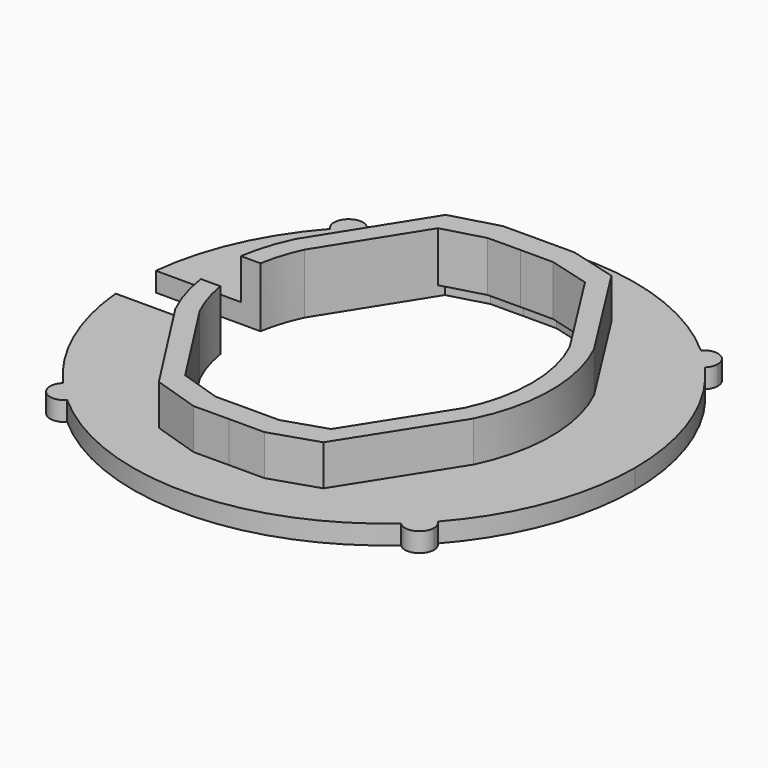
from build123d import *

# Parameters (mm, degrees)
F1_DEPTH = 3.1
F3_DEPTH = 1
F5_DEPTH = 3.1
F7_DEPTH = 2.6


# Not quite as in the source:
# - ends of sketch curves that miss each other by under 0.0002 mm in the source are joined


with BuildPart() as f1:
    # F0 (on Top) → F1 (new body)
    with BuildSketch(Plane.XY):
        with BuildLine():
            Line((-45.1821846682, -49.2377741688), (-48.6372292437, -43.7981166044))
            Line((-48.6372292437, -43.7981166044), (-51.0690886894, -43.1337059986))
            Line((-51.0690886894, -43.1337059986), (-52.9226313652, -43.1337059986))
            Line((-52.9226313652, -43.1337059986), (-54.7761512226, -43.1429032238))
            Line((-54.7761512226, -43.1429032238), (-57.2046839443, -43.8193724666))
            Line((-57.2046839443, -43.8193724666), (-60.6326945623, -49.2761068966))
            ThreePointArc((-60.6326945623, -49.2761068966), (-61.5175196788, -53.1892877339), (-60.5939044307, -57.0934950318))
            Line((-60.5939044307, -57.0934950318), (-57.1270457212, -62.4923727119))
            Line((-57.1270457212, -62.4923727119), (-54.7013924586, -63.2718429691))
            Line((-54.7013924586, -63.2718429691), (-52.8726911435, -63.2627688943))
            Line((-52.8726911435, -63.2627688943), (-51.0439673156, -63.2627688943))
            Line((-51.0439673156, -63.2627688943), (-48.6222116233, -62.4712722115))
            Line((-48.6222116233, -62.4712722115), (-45.1821846682, -57.0552585424))
            ThreePointArc((-45.1821846682, -57.0552585424), (-44.2779533541, -53.1465163556), (-45.1821846682, -49.2377741688))
        make_face()
        with BuildLine():
            Line((-51.2032357795, -44.1337052485), (-49.2739452053, -44.6608085404))
            Line((-49.2739452053, -44.6608085404), (-46.0570379398, -49.725540285))
            ThreePointArc((-46.0570379398, -49.725540285), (-45.277952604, -53.1465163556), (-46.0570379398, -56.5674924262))
            Line((-46.0570379398, -56.5674924262), (-49.2739452053, -61.6322241709))
            Line((-49.2739452053, -61.6322241709), (-51.2032357795, -62.2627696444))
            Line((-51.2032357795, -62.2627696444), (-52.8751721425, -62.2627696444))
            Line((-52.8751721425, -62.2627696444), (-54.5470879228, -62.2710657443))
            Line((-54.5470879228, -62.2710657443), (-56.4794834946, -61.6501011173))
            Line((-56.4794834946, -61.6501011173), (-59.7214822105, -56.6013939237))
            ThreePointArc((-59.7214822105, -56.6013939237), (-60.5175327396, -53.1843257665), (-59.7554317793, -49.7595260114))
            Line((-59.7554317793, -49.7595260114), (-56.5636951686, -44.678894416))
            Line((-56.5636951686, -44.678894416), (-54.6370438166, -44.1422245291))
            Line((-54.6370438166, -44.1422245291), (-52.9201503662, -44.1337052485))
            Line((-52.9201503662, -44.1337052485), (-51.2032357795, -44.1337052485))
        make_face(mode=Mode.SUBTRACT)
    extrude(amount=F1_DEPTH)

    # F2 (on face) → F3 (join)
    with BuildSketch(Plane(origin=(0, 0, 0), x_dir=(1, 0, 0), z_dir=(0, 0, -1))):
        with BuildLine():
            ThreePointArc((-43.358584194, 62.0303384897), (-43.2740778057, 61.9381826183), (-43.1904616862, 61.8452182226))
            ThreePointArc((-43.1904616862, 61.8452182226), (-43.0165755747, 62.0936479592), (-42.9552730989, 62.3906256019))
            ThreePointArc((-42.9552730989, 62.3906256019), (-43.4282853143, 63.0876031964), (-44.2506804781, 62.9054370146))
            ThreePointArc((-44.2506804781, 62.9054370146), (-44.1577160825, 62.8218208951), (-44.0655602111, 62.7373145068))
            ThreePointArc((-44.0655602111, 62.7373145068), (-43.5183821629, 62.8543839205), (-43.2052730989, 62.3906256019))
            ThreePointArc((-43.2052730989, 62.3906256019), (-43.2451945988, 62.1948507981), (-43.358584194, 62.0303384897))
        make_face()
        with BuildLine():
            ThreePointArc((-44.0655602111, 62.7373145068), (-43.7052730989, 62.3906256019), (-43.358584194, 62.0303384897))
            ThreePointArc((-43.358584194, 62.0303384897), (-43.2451945988, 62.1948507981), (-43.2052730989, 62.3906256019))
            ThreePointArc((-43.2052730989, 62.3906256019), (-43.5183821629, 62.8543839205), (-44.0655602111, 62.7373145068))
        make_face()
        with BuildLine():
            ThreePointArc((-44.0655602111, 62.7373145068), (-44.0588264895, 62.0370722113), (-43.358584194, 62.0303384897))
            ThreePointArc((-43.358584194, 62.0303384897), (-43.7052730989, 62.3906256019), (-44.0655602111, 62.7373145068))
        make_face()
        with BuildLine():
            ThreePointArc((-43.1904616862, 44.5512566703), (-40.748719029, 48.5718778834), (-39.8976612543, 53.1982374465))
            ThreePointArc((-39.8976612543, 53.1982374465), (-40.748719029, 57.8245970095), (-43.1904616862, 61.8452182226))
            ThreePointArc((-43.1904616862, 61.8452182226), (-44.2356031848, 61.860295516), (-44.2506804781, 62.9054370146))
            ThreePointArc((-44.2506804781, 62.9054370146), (-52.8976612543, 66.1982374465), (-61.5446420305, 62.9054370146))
            ThreePointArc((-61.5446420305, 62.9054370146), (-61.3930718153, 62.6676133864), (-61.3400494097, 62.3906256019))
            ThreePointArc((-61.3400494097, 62.3906256019), (-61.7930717671, 61.7019280777), (-62.6048608225, 61.8452182226))
            ThreePointArc((-62.6048608225, 61.8452182226), (-65.8976612543, 53.1982374465), (-62.6048608225, 44.5512566703))
            ThreePointArc((-62.6048608225, 44.5512566703), (-61.7930717671, 44.6945468152), (-61.3400494097, 44.005849291))
            ThreePointArc((-61.3400494097, 44.005849291), (-61.3930718153, 43.7288615065), (-61.5446420305, 43.4910378783))
            ThreePointArc((-61.5446420305, 43.4910378783), (-52.8976612543, 40.1982374465), (-44.2506804781, 43.4910378783))
            ThreePointArc((-44.2506804781, 43.4910378783), (-44.2356031848, 44.5361793769), (-43.1904616862, 44.5512566703))
        make_face()
        with BuildLine():
            Line((-45.1821846682, 49.2377741688), (-48.6372292437, 43.7981166044))
            Line((-48.6372292437, 43.7981166044), (-51.0690886894, 43.1337059986))
            Line((-51.0690886894, 43.1337059986), (-52.9226313652, 43.1337059986))
            Line((-52.9226313652, 43.1337059986), (-54.7761512226, 43.1429032238))
            Line((-54.7761512226, 43.1429032238), (-57.2046839443, 43.8193724666))
            Line((-57.2046839443, 43.8193724666), (-60.6326945623, 49.2761068966))
            ThreePointArc((-60.6326945623, 49.2761068966), (-61.5175196788, 53.1892877339), (-60.5939044307, 57.0934950318))
            Line((-60.5939044307, 57.0934950318), (-57.1270457212, 62.4923727119))
            Line((-57.1270457212, 62.4923727119), (-54.7013924586, 63.2718429691))
            Line((-54.7013924586, 63.2718429691), (-52.8726911435, 63.2627688943))
            Line((-52.8726911435, 63.2627688943), (-51.0439673156, 63.2627688943))
            Line((-51.0439673156, 63.2627688943), (-48.6222116233, 62.4712722115))
            Line((-48.6222116233, 62.4712722115), (-45.1821846682, 57.0552585424))
            ThreePointArc((-45.1821846682, 57.0552585424), (-44.2779533541, 53.1465163556), (-45.1821846682, 49.2377741688))
        make_face(mode=Mode.SUBTRACT)
        with BuildLine():
            ThreePointArc((-44.2506804781, 62.9054370146), (-44.2356031848, 61.860295516), (-43.1904616862, 61.8452182226))
            ThreePointArc((-43.1904616862, 61.8452182226), (-43.2740778057, 61.9381826183), (-43.358584194, 62.0303384897))
            ThreePointArc((-43.358584194, 62.0303384897), (-44.0588264895, 62.0370722113), (-44.0655602111, 62.7373145068))
            ThreePointArc((-44.0655602111, 62.7373145068), (-44.1577160825, 62.8218208951), (-44.2506804781, 62.9054370146))
        make_face()
        with BuildLine():
            ThreePointArc((-61.7297622975, 62.7373145068), (-61.6376064262, 62.8218208951), (-61.5446420305, 62.9054370146))
            ThreePointArc((-61.5446420305, 62.9054370146), (-62.6203794956, 62.9209556878), (-62.6048608225, 61.8452182226))
            ThreePointArc((-62.6048608225, 61.8452182226), (-62.521244703, 61.9381826183), (-62.4367383146, 62.0303384897))
            ThreePointArc((-62.4367383146, 62.0303384897), (-62.4436028003, 62.7441789925), (-61.7297622975, 62.7373145068))
        make_face()
        with BuildLine():
            ThreePointArc((-61.3400494097, 62.3906256019), (-61.3930718153, 62.6676133864), (-61.5446420305, 62.9054370146))
            ThreePointArc((-61.5446420305, 62.9054370146), (-61.6376064262, 62.8218208951), (-61.7297622975, 62.7373145068))
            ThreePointArc((-61.7297622975, 62.7373145068), (-61.6262910912, 62.5775165378), (-61.5900494097, 62.3906256019))
            ThreePointArc((-61.5900494097, 62.3906256019), (-61.894274606, 61.9305471018), (-62.4367383146, 62.0303384897))
            ThreePointArc((-62.4367383146, 62.0303384897), (-62.521244703, 61.9381826183), (-62.6048608225, 61.8452182226))
            ThreePointArc((-62.6048608225, 61.8452182226), (-61.7930717671, 61.7019280777), (-61.3400494097, 62.3906256019))
        make_face()
        with BuildLine():
            ThreePointArc((-62.4367383146, 62.0303384897), (-62.0900494097, 62.3906256019), (-61.7297622975, 62.7373145068))
            ThreePointArc((-61.7297622975, 62.7373145068), (-62.4436028003, 62.7441789925), (-62.4367383146, 62.0303384897))
        make_face()
        with BuildLine():
            ThreePointArc((-61.5900494097, 62.3906256019), (-61.6262910912, 62.5775165378), (-61.7297622975, 62.7373145068))
            ThreePointArc((-61.7297622975, 62.7373145068), (-62.0900494097, 62.3906256019), (-62.4367383146, 62.0303384897))
            ThreePointArc((-62.4367383146, 62.0303384897), (-61.894274606, 61.9305471018), (-61.5900494097, 62.3906256019))
        make_face()
        with BuildLine():
            ThreePointArc((-42.9552730989, 44.005849291), (-43.0165755747, 44.3028269337), (-43.1904616862, 44.5512566703))
            ThreePointArc((-43.1904616862, 44.5512566703), (-43.2740778057, 44.4582922746), (-43.358584194, 44.3661364032))
            ThreePointArc((-43.358584194, 44.3661364032), (-43.2451945988, 44.2016240948), (-43.2052730989, 44.005849291))
            ThreePointArc((-43.2052730989, 44.005849291), (-43.5183821629, 43.5420909724), (-44.0655602111, 43.6591603861))
            ThreePointArc((-44.0655602111, 43.6591603861), (-44.1577160825, 43.5746539978), (-44.2506804781, 43.4910378783))
            ThreePointArc((-44.2506804781, 43.4910378783), (-43.4282853143, 43.3088716965), (-42.9552730989, 44.005849291))
        make_face()
        with BuildLine():
            ThreePointArc((-43.2052730989, 44.005849291), (-43.2451945988, 44.2016240948), (-43.358584194, 44.3661364032))
            ThreePointArc((-43.358584194, 44.3661364032), (-43.7052730989, 44.005849291), (-44.0655602111, 43.6591603861))
            ThreePointArc((-44.0655602111, 43.6591603861), (-43.5183821629, 43.5420909724), (-43.2052730989, 44.005849291))
        make_face()
        with BuildLine():
            ThreePointArc((-44.0655602111, 43.6591603861), (-43.7052730989, 44.005849291), (-43.358584194, 44.3661364032))
            ThreePointArc((-43.358584194, 44.3661364032), (-44.0588264895, 44.3594026816), (-44.0655602111, 43.6591603861))
        make_face()
        with BuildLine():
            ThreePointArc((-43.358584194, 44.3661364032), (-43.2740778057, 44.4582922746), (-43.1904616862, 44.5512566703))
            ThreePointArc((-43.1904616862, 44.5512566703), (-44.2356031848, 44.5361793769), (-44.2506804781, 43.4910378783))
            ThreePointArc((-44.2506804781, 43.4910378783), (-44.1577160825, 43.5746539978), (-44.0655602111, 43.6591603861))
            ThreePointArc((-44.0655602111, 43.6591603861), (-44.0588264895, 44.3594026816), (-43.358584194, 44.3661364032))
        make_face()
        with BuildLine():
            ThreePointArc((-62.6048608225, 44.5512566703), (-62.6203794956, 43.4755192051), (-61.5446420305, 43.4910378783))
            ThreePointArc((-61.5446420305, 43.4910378783), (-61.6376064262, 43.5746539978), (-61.7297622975, 43.6591603861))
            ThreePointArc((-61.7297622975, 43.6591603861), (-62.4436028003, 43.6522959004), (-62.4367383146, 44.3661364032))
            ThreePointArc((-62.4367383146, 44.3661364032), (-62.521244703, 44.4582922746), (-62.6048608225, 44.5512566703))
        make_face()
        with BuildLine():
            ThreePointArc((-62.4367383146, 44.3661364032), (-62.4436028003, 43.6522959004), (-61.7297622975, 43.6591603861))
            ThreePointArc((-61.7297622975, 43.6591603861), (-62.0900494097, 44.005849291), (-62.4367383146, 44.3661364032))
        make_face()
        with BuildLine():
            ThreePointArc((-62.4367383146, 44.3661364032), (-62.0900494097, 44.005849291), (-61.7297622975, 43.6591603861))
            ThreePointArc((-61.7297622975, 43.6591603861), (-61.6262910912, 43.8189583551), (-61.5900494097, 44.005849291))
            ThreePointArc((-61.5900494097, 44.005849291), (-61.894274606, 44.4659277911), (-62.4367383146, 44.3661364032))
        make_face()
        with BuildLine():
            ThreePointArc((-61.7297622975, 43.6591603861), (-61.6376064262, 43.5746539978), (-61.5446420305, 43.4910378783))
            ThreePointArc((-61.5446420305, 43.4910378783), (-61.3930718153, 43.7288615065), (-61.3400494097, 44.005849291))
            ThreePointArc((-61.3400494097, 44.005849291), (-61.7930717671, 44.6945468152), (-62.6048608225, 44.5512566703))
            ThreePointArc((-62.6048608225, 44.5512566703), (-62.521244703, 44.4582922746), (-62.4367383146, 44.3661364032))
            ThreePointArc((-62.4367383146, 44.3661364032), (-61.894274606, 44.4659277911), (-61.5900494097, 44.005849291))
            ThreePointArc((-61.5900494097, 44.005849291), (-61.6262910912, 43.8189583551), (-61.7297622975, 43.6591603861))
        make_face()
    extrude(amount=-F3_DEPTH)

    # F4 (on face) → F5 (cut)
    with BuildSketch(Plane(origin=(0, 0, 0), x_dir=(1, 0, 0), z_dir=(0, 0, -1))):
        with BuildLine():
            Line((-60.4180157971, 54.3957427144), (-65.8423891824, 54.3957427144))
            ThreePointArc((-65.8423891824, 54.3957427144), (-65.8973302268, 53.1054656449), (-65.8239796584, 51.8161041253))
            Line((-65.8239796584, 51.8161041253), (-60.4050414596, 51.8161041253))
            ThreePointArc((-60.4050414596, 51.8161041253), (-60.5175300761, 53.1053902837), (-60.4180157971, 54.3957427144))
        make_face()
    extrude(amount=-F5_DEPTH, mode=Mode.SUBTRACT)

    # F6 (on face) → F7 (join)
    with BuildSketch(Plane.XY.offset(3.1)):
        Polygon((-56.5636951686, -44.678894416), (-56.7217861266, -44.930544854), (-54.6092223145, -44.34208894), (-52.920150354, -44.3337077106), (-52.919157972, -44.3337027864), (-51.2300652176, -44.3337052485), (-49.1146075113, -44.9116714376), (-49.2739452053, -44.6608085404), (-51.2032357795, -44.1337052485), (-52.9201503662, -44.1337052485), (-54.6370438166, -44.1422245291), align=None)
        Polygon((-49.2739452053, -61.6322241709), (-49.1052905017, -61.3666924783), (-51.2350894961, -62.0627696444), (-52.8756683426, -62.0627696444), (-54.5162269925, -62.0709101492), (-56.6494536825, -61.3854095534), (-56.4794834946, -61.6501011173), (-54.5470879228, -62.2710657443), (-52.8751721425, -62.2627696444), (-51.2032357795, -62.2627696444), align=None)
    extrude(amount=-F7_DEPTH)


solid = f1.part
